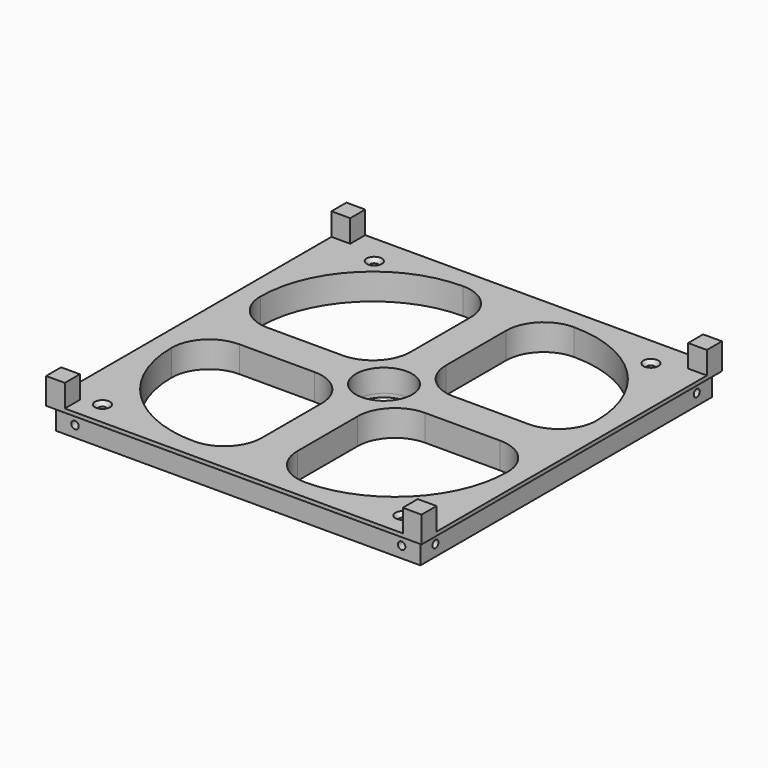
from build123d import *

# Parameters (mm, degrees)
F0_W            = 97
F0_H            = 97
F0_R            = 7.4829182058
F1_DEPTH        = 6
F0_W_2          = 100
F0_H_2          = 100
F1_FACE_W       = 97
F1_FACE_H       = 97
F1_FACE_R       = 7.4829182058
F2_DEPTH        = 1
F4_D            = 2
F4_DEPTH        = 20
F4_TIP          = 0.600860619
F6_D            = 2
F6_DEPTH        = 20
F6_TIP          = 0.600860619
F8_D            = 2
F8_DEPTH        = 20
F8_TIP          = 0.600860619
F10_D           = 2
F10_DEPTH       = 20
F10_TIP         = 0.600860619
F12_D           = 2
F12_CSINK_D     = 4
F12_CSINK_ANGLE = 90
F11_W           = 5
F11_H           = 5
F13_DEPTH       = 6


with BuildPart() as f1:
    # F0 (on Top) → F1 (new body)
    with BuildSketch(Plane.XY):
        Rectangle(F0_W, F0_H)
        with BuildLine():
            ThreePointArc((-14.75, -4.75), (-7.6789321881, -7.6789321881), (-4.75, -14.75))
            Line((-4.75, -14.75), (-4.75, -34.75))
            ThreePointArc((-4.75, -34.75), (-7.6789321881, -41.8210678119), (-14.75, -44.75))
            ThreePointArc((-14.75, -44.75), (-35.9632034356, -35.9632034356), (-44.75, -14.75))
            ThreePointArc((-44.75, -14.75), (-41.8210678119, -7.6789321881), (-34.75, -4.75))
            Line((-34.75, -4.75), (-14.75, -4.75))
        make_face(mode=Mode.SUBTRACT)
        with BuildLine():
            ThreePointArc((4.75, -14.75), (7.6789321881, -7.6789321881), (14.75, -4.75))
            Line((14.75, -4.75), (34.75, -4.75))
            ThreePointArc((34.75, -4.75), (41.8210678119, -7.6789321881), (44.75, -14.75))
            ThreePointArc((44.75, -14.75), (35.9632034356, -35.9632034356), (14.75, -44.75))
            ThreePointArc((14.75, -44.75), (7.6789321881, -41.8210678119), (4.75, -34.75))
            Line((4.75, -34.75), (4.75, -14.75))
        make_face(mode=Mode.SUBTRACT)
        with BuildLine():
            ThreePointArc((-4.75, 14.75), (-7.6789321881, 7.6789321881), (-14.75, 4.75))
            Line((-14.75, 4.75), (-34.75, 4.75))
            ThreePointArc((-34.75, 4.75), (-41.8210678119, 7.6789321881), (-44.75, 14.75))
            ThreePointArc((-44.75, 14.75), (-35.9632034356, 35.9632034356), (-14.75, 44.75))
            ThreePointArc((-14.75, 44.75), (-7.6789321881, 41.8210678119), (-4.75, 34.75))
            Line((-4.75, 34.75), (-4.75, 14.75))
        make_face(mode=Mode.SUBTRACT)
        Circle(F0_R, mode=Mode.SUBTRACT)
        with BuildLine():
            ThreePointArc((14.75, 4.75), (7.6789321881, 7.6789321881), (4.75, 14.75))
            Line((4.75, 14.75), (4.75, 34.75))
            ThreePointArc((4.75, 34.75), (7.6789321881, 41.8210678119), (14.75, 44.75))
            ThreePointArc((14.75, 44.75), (35.9632034356, 35.9632034356), (44.75, 14.75))
            ThreePointArc((44.75, 14.75), (41.8210678119, 7.6789321881), (34.75, 4.75))
            Line((34.75, 4.75), (14.75, 4.75))
        make_face(mode=Mode.SUBTRACT)
    extrude(amount=-F1_DEPTH)

    # F0 (on Top) + F1_face (on face) → F2 (join)
    with BuildSketch(Plane.XY):
        Rectangle(F0_W_2, F0_H_2)
        Rectangle(F0_W, F0_H, mode=Mode.SUBTRACT)
    with BuildSketch(Plane(origin=(0, 0, -6), x_dir=(1, 0, 0), z_dir=(0, 0, -1))):
        Rectangle(F1_FACE_W, F1_FACE_H)
        with BuildLine():
            ThreePointArc((-34.75, 4.75), (-41.8210678119, 7.6789321881), (-44.75, 14.75))
            ThreePointArc((-44.75, 14.75), (-35.9632034356, 35.9632034356), (-14.75, 44.75))
            ThreePointArc((-14.75, 44.75), (-7.6789321881, 41.8210678119), (-4.75, 34.75))
            Line((-4.75, 34.75), (-4.75, 14.75))
            ThreePointArc((-4.75, 14.75), (-7.6789321881, 7.6789321881), (-14.75, 4.75))
            Line((-14.75, 4.75), (-34.75, 4.75))
        make_face(mode=Mode.SUBTRACT)
        with BuildLine():
            ThreePointArc((14.75, 4.75), (7.6789321881, 7.6789321881), (4.75, 14.75))
            Line((4.75, 14.75), (4.75, 34.75))
            ThreePointArc((4.75, 34.75), (7.6789321881, 41.8210678119), (14.75, 44.75))
            ThreePointArc((14.75, 44.75), (35.9632034356, 35.9632034356), (44.75, 14.75))
            ThreePointArc((44.75, 14.75), (41.8210678119, 7.6789321881), (34.75, 4.75))
            Line((34.75, 4.75), (14.75, 4.75))
        make_face(mode=Mode.SUBTRACT)
        with BuildLine():
            ThreePointArc((-14.75, -4.75), (-7.6789321881, -7.6789321881), (-4.75, -14.75))
            Line((-4.75, -14.75), (-4.75, -34.75))
            ThreePointArc((-4.75, -34.75), (-7.6789321881, -41.8210678119), (-14.75, -44.75))
            ThreePointArc((-14.75, -44.75), (-35.9632034356, -35.9632034356), (-44.75, -14.75))
            ThreePointArc((-44.75, -14.75), (-41.8210678119, -7.6789321881), (-34.75, -4.75))
            Line((-34.75, -4.75), (-14.75, -4.75))
        make_face(mode=Mode.SUBTRACT)
        Circle(F1_FACE_R, mode=Mode.SUBTRACT)
        with BuildLine():
            ThreePointArc((34.75, -4.75), (41.8210678119, -7.6789321881), (44.75, -14.75))
            ThreePointArc((44.75, -14.75), (35.9632034356, -35.9632034356), (14.75, -44.75))
            ThreePointArc((14.75, -44.75), (7.6789321881, -41.8210678119), (4.75, -34.75))
            Line((4.75, -34.75), (4.75, -14.75))
            ThreePointArc((4.75, -14.75), (7.6789321881, -7.6789321881), (14.75, -4.75))
            Line((14.75, -4.75), (34.75, -4.75))
        make_face(mode=Mode.SUBTRACT)
    extrude(amount=-F2_DEPTH, dir=(0, 0, 1))

    # F4
    with Locations(Plane(origin=(0, 48.5, 0), x_dir=(-1, 0, 0), z_dir=(0, 1, 0))):
        with Locations((-43.5, -4), (43.5, -4)):
            Hole(F4_D / 2, depth=F4_DEPTH)
            with Locations((0, 0, -(F4_DEPTH + F4_TIP / 2))):  # 118° drill point
                Cone(0, F4_D / 2, F4_TIP, mode=Mode.SUBTRACT)

    # F6
    with Locations(Plane(origin=(-48.5, 0, 0), x_dir=(0, -1, 0), z_dir=(-1, 0, 0))):
        with Locations((-43.5, -4), (43.5, -4)):
            Hole(F6_D / 2, depth=F6_DEPTH)
            with Locations((0, 0, -(F6_DEPTH + F6_TIP / 2))):  # 118° drill point
                Cone(0, F6_D / 2, F6_TIP, mode=Mode.SUBTRACT)

    # F8
    with Locations(Plane.XZ.offset(48.5)):
        with Locations((-43.5, -4), (43.5, -4)):
            Hole(F8_D / 2, depth=F8_DEPTH)
            with Locations((0, 0, -(F8_DEPTH + F8_TIP / 2))):  # 118° drill point
                Cone(0, F8_D / 2, F8_TIP, mode=Mode.SUBTRACT)

    # F10
    with Locations(Plane.YZ.offset(48.5)):
        with Locations((-43.5, -4), (43.5, -4)):
            Hole(F10_D / 2, depth=F10_DEPTH)
            with Locations((0, 0, -(F10_DEPTH + F10_TIP / 2))):  # 118° drill point
                Cone(0, F10_D / 2, F10_TIP, mode=Mode.SUBTRACT)

    # F12 (through all)
    with Locations(Plane.XY):
        with Locations((37.465, 42.011), (-36.195, 42.011), (40.005, -43.7191091478), (-40.005, -43.7191091478)):
            CounterSinkHole(F12_D / 2, F12_CSINK_D / 2, counter_sink_angle=F12_CSINK_ANGLE)

    # F11 (on face) → F13 (join)
    with BuildSketch(Plane.XY):
        with Locations((47.5, 47.5)):
            Rectangle(F11_W, F11_H)
        with Locations((47.5, -47.5)):
            Rectangle(F11_W, F11_H)
        with Locations((-47.5, -47.5)):
            Rectangle(F11_W, F11_H)
        with Locations((-47.5, 47.5)):
            Rectangle(F11_W, F11_H)
    extrude(amount=F13_DEPTH)


solid = f1.part
